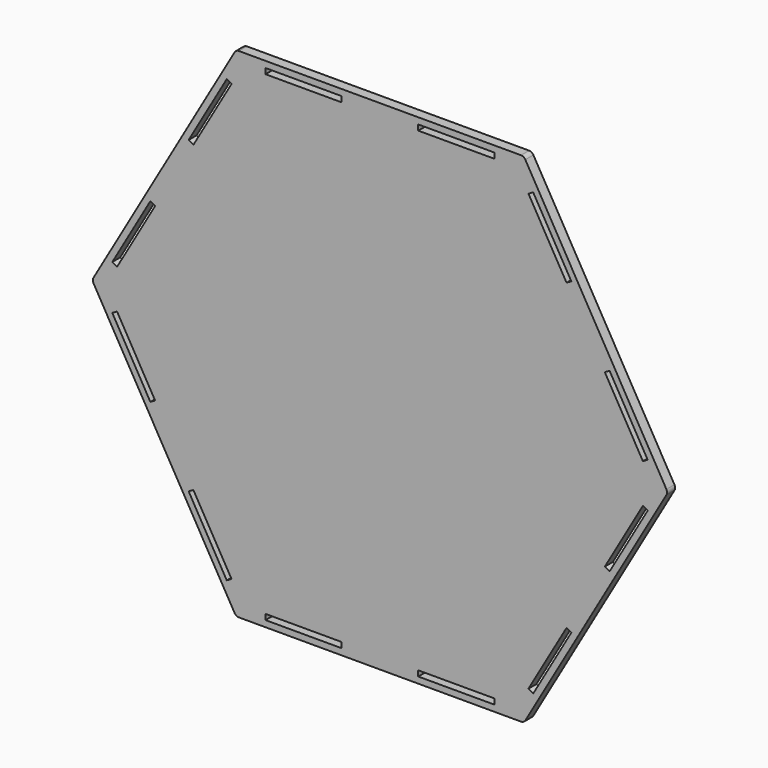
from build123d import *

# Parameters (mm, degrees)
F1_DEPTH        = 5.08
F2_W            = 38.4310525078
F2_H            = 2.7686
F3_DEPTH        = 5.08
F3_COPIES_COUNT = 6


# Not quite as in the source:
# - a pattern or mirror of a feature is missing from the dataset's text; its kind, count and spacing are read off the source's solid


with BuildPart() as f1:
    # F0 (on Front) → F1 (new body)
    with BuildSketch(Plane.XZ):
        with BuildLine():
            Line((71.1237796615, 125.73), (-71.1237796615, 125.73))
            ThreePointArc((-71.1237796615, 125.73), (-72.3937796615, 125.3897045256), (-73.3234841871, 124.46))
            Line((-73.3234841871, 124.46), (-144.4472638486, 1.27))
            ThreePointArc((-144.4472638486, 1.27), (-144.7875593229, 0), (-144.4472638486, -1.27))
            Line((-144.4472638486, -1.27), (-73.3234841871, -124.46))
            ThreePointArc((-73.3234841871, -124.46), (-72.3937796615, -125.3897045256), (-71.1237796615, -125.73))
            Line((-71.1237796615, -125.73), (71.1237796615, -125.73))
            ThreePointArc((71.1237796615, -125.73), (72.3937796615, -125.3897045256), (73.3234841871, -124.46))
            Line((73.3234841871, -124.46), (144.4472638486, -1.27))
            ThreePointArc((144.4472638486, -1.27), (144.7875593229, 0), (144.4472638486, 1.27))
            Line((144.4472638486, 1.27), (73.3234841871, 124.46))
            ThreePointArc((73.3234841871, 124.46), (72.3937796615, 125.3897045256), (71.1237796615, 125.73))
        make_face()
    extrude(amount=F1_DEPTH)

    # F2 (on face) → F3 (cut, through all)
    with BuildSketch(Plane.XZ.offset(5.08)):
        with Locations((-38.5195262539, 121.1707)):
            Rectangle(F2_W, F2_H)
        with Locations((38.5195262539, 121.1707)):
            Rectangle(F2_W, F2_H)
    f3 = extrude(amount=-F3_DEPTH, mode=Mode.SUBTRACT)

    # F3_copies: F3 ×6 about axis
    f3_copies_axis = Axis((0, 0, 0), (0, 1, 0))
    for i in range(1, F3_COPIES_COUNT):
        add(f3.rotate(f3_copies_axis, i * 360 / F3_COPIES_COUNT), mode=Mode.SUBTRACT)


solid = f1.part
